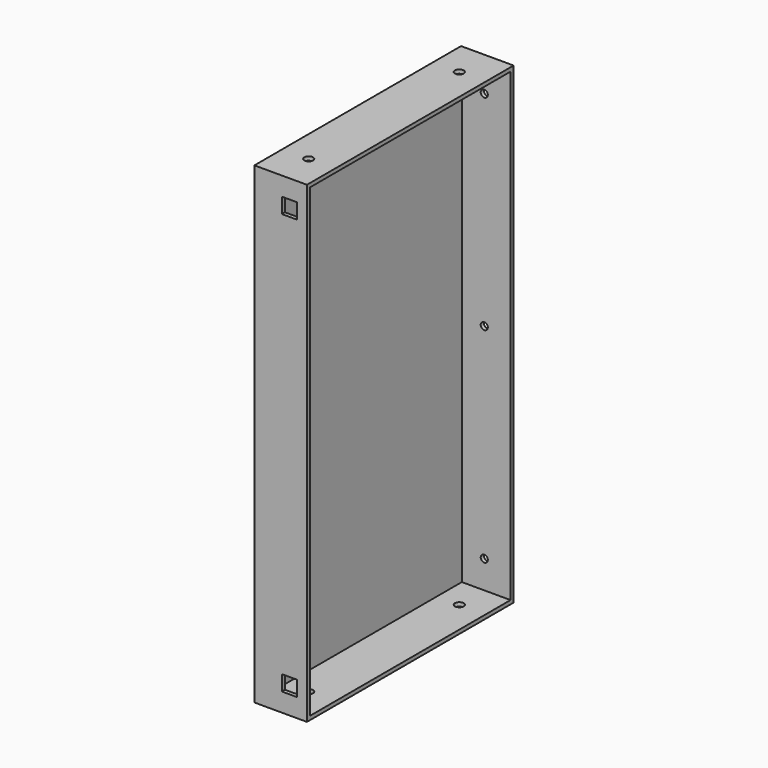
from build123d import *

# Parameters (mm, degrees)
F0_W     = 38.1
F0_H     = 187.325
F1_DEPTH = 171.45
F2_T     = -2.778125
F3_R     = 2.5796875
F4_DEPTH = 2.778125
F5_R     = 3.175
F6_DEPTH = 342.901
F7_W     = 11.1125
F7_H     = 11.1125
F8_DEPTH = 2.778125


# Not quite as in the source:
# - a feature names something its author has since deleted; it is built from what else it names


with BuildPart() as f1:
    # F0 (on Top) → F1 (new body, symmetric)
    with BuildSketch(Plane.XY):
        with Locations((19.05, 93.6625)):
            Rectangle(F0_W, F0_H)
    extrude(amount=F1_DEPTH, both=True)

    # F2
    f2_openings = [f1.faces().sort_by_distance(p)[0] for p in [
        (38.1, 93.6625, 0),
    ]]
    offset(amount=F2_T, openings=f2_openings)

    # F3 (on face) → F4 (cut, through all)
    with BuildSketch(Plane(origin=(0, 187.325, 0), x_dir=(-1, 0, 0), z_dir=(0, 1, 0))):
        with Locations((-19.05, 148.43125)):
            Circle(F3_R)
        with Locations((-19.05, 0)):
            Circle(F3_R)
        with Locations((-19.05, -148.43125)):
            Circle(F3_R)
    extrude(amount=-F4_DEPTH, mode=Mode.SUBTRACT)

    # F5 (on face) → F6 (cut, through all)
    with BuildSketch(Plane.XY.offset(171.45)):
        with Locations((19.05, 161.925)):
            Circle(F5_R)
        with Locations((19.05, 25.4)):
            Circle(F5_R)
    extrude(amount=-F6_DEPTH, mode=Mode.SUBTRACT)

    # F7 (on face) → F8 (cut, through all)
    with BuildSketch(Plane.XZ):
        with Locations((25.4, 152.4)):
            Rectangle(F7_W, F7_H)
        with Locations((25.4, -152.4)):
            Rectangle(F7_W, F7_H)
    extrude(amount=-F8_DEPTH, mode=Mode.SUBTRACT)


solid = f1.part
